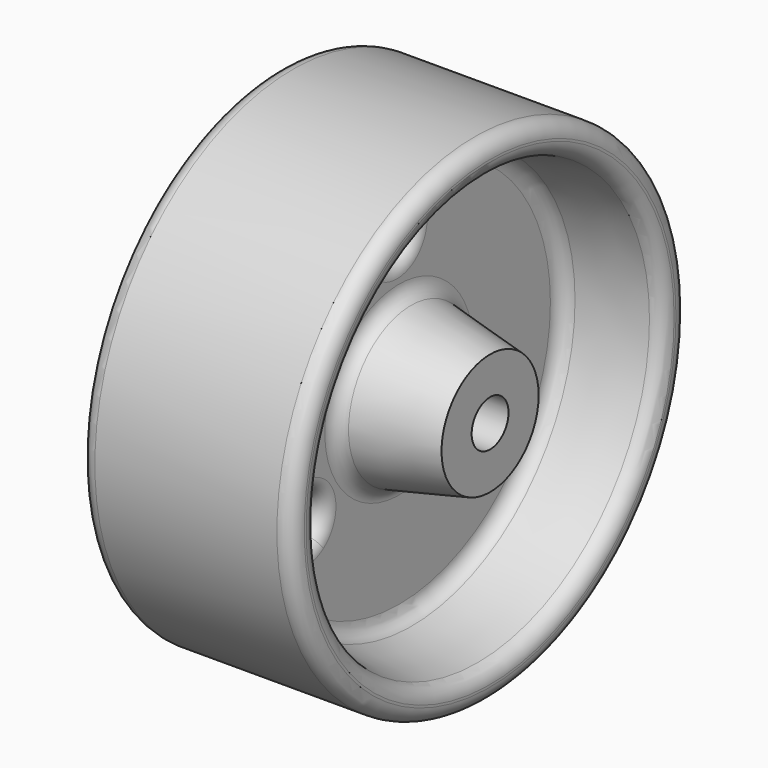
from build123d import *

# Parameters (mm, degrees)
F2_R     = 3.175
F4_DEPTH = 25.4
F5_R     = 3.17499


# Not quite as in the source:
# - a fillet or chamfer is up to 0.001 mm smaller than in the source, because OpenCascade refuses the exact size


with BuildPart() as f1:
    # F0 (on Top) → F1 (revolve)
    with BuildSketch(Plane.XY):
        Polygon((-25.8535725378, 7.874), (-25.8535725378, 0), (24.9464274622, 0), (24.9464274622, 7.874), (5.8964274622, 12.0600205039), (-0.4535725378, 12.0600205039), align=None)
        Polygon((-0.4535725378, 37.4600205039), (-0.4535725378, 12.0600205039), (5.8964274622, 12.0600205039), (5.8964274622, 37.4600205039), (24.9464274622, 40.6350205039), (24.9464274622, 46.9850205039), (-0.4535725378, 46.9850205039), align=None)
        Polygon((-19.5035725378, 40.6350205039), (-0.4535725378, 37.4600205039), (-0.4535725378, 46.9850205039), (-19.5035725378, 46.9850205039), align=None)
    revolve(axis=Axis((-0.2934029948, -4.826, 0), (1, 0, 0)))

    # F2
    f2_edges = [f1.edges().sort_by_distance(p)[0] for p in [
        (5.896427, -47.112021, 0),
        (24.946427, -50.287021, 0),
        (24.946427, -56.637021, 0),
        (5.896427, -21.712021, 0),
        (-19.503573, -56.637021, 0),
        (-19.503573, -50.287021, 0),
        (-0.453573, -21.712021, 0),
        (-0.453573, -47.112021, 0),
    ]]
    fillet(f2_edges, radius=F2_R)

    # F3 (on face) → F4 (cut)
    with BuildSketch(Plane(origin=(-0.4535725378, 0, 0), x_dir=(0, -1, 0), z_dir=(-1, 0, 0))):
        with BuildLine():
            ThreePointArc((0.658709515, 28.2694944244), (5.314152326, 23.8074959531), (10.1485843232, 28.0749126646))
            ThreePointArc((10.1485843232, 28.0749126646), (5.4117827912, 28.5689951437), (0.658709515, 28.2694944244))
        make_face()
        with BuildLine():
            ThreePointArc((0.658709515, 28.2694944244), (5.4117827912, 28.5689951437), (10.1485843232, 28.0749126646))
            ThreePointArc((10.1485843232, 28.0749126646), (10.1678538349, 28.3216199694), (10.1742827912, 28.5689951437))
            ThreePointArc((10.1742827912, 28.5689951437), (5.2619582739, 33.3291378794), (0.658709515, 28.2694944244))
        make_face()
        with BuildLine():
            ThreePointArc((34.0370841595, -14.7918003501), (33.3220764355, -12.2819771442), (31.3917455662, -10.5257677872))
            ThreePointArc((31.3917455662, -10.5257677872), (29.2745841595, -14.7918003501), (26.4782954149, -18.64694957))
            ThreePointArc((26.4782954149, -18.64694957), (31.4383864961, -19.0343662834), (34.0370841595, -14.7918003501))
        make_face()
        with BuildLine():
            ThreePointArc((26.4782954149, -18.64694957), (29.2745841595, -14.7918003501), (31.3917455662, -10.5257677872))
            ThreePointArc((31.3917455662, -10.5257677872), (25.1998201329, -12.3265002918), (26.4782954149, -18.64694957))
        make_face()
        with BuildLine():
            ThreePointArc((-15.4458669506, -13.7771947936), (-17.6160982435, -9.7820040347), (-22.1488797381, -9.4279630946))
            ThreePointArc((-22.1488797381, -9.4279630946), (-20.2083669506, -13.7771947936), (-17.5724550812, -17.7437266372))
            ThreePointArc((-17.5724550812, -17.7437266372), (-16.0110501572, -16.0275143233), (-15.4458669506, -13.7771947936))
        make_face()
        with BuildLine():
            ThreePointArc((-17.5724550812, -17.7437266372), (-20.2083669506, -13.7771947936), (-22.1488797381, -9.4279630946))
            ThreePointArc((-22.1488797381, -9.4279630946), (-24.3807614424, -16.0733939259), (-17.5724550812, -17.7437266372))
        make_face()
    extrude(amount=-F4_DEPTH, mode=Mode.SUBTRACT)

    # F5 (radius 3.175 in the source; OpenCascade refuses exactly that, so slightly less here)
    f5_edges = [f1.edges().sort_by_distance(p)[0] for p in [
        (-0.453573, 18.267854, -18.126426),
        (5.896427, 18.267854, -18.126426),
        (-0.453573, -27.157423, -19.057833),
        (5.896427, -27.157423, -19.057833),
        (-0.453573, -0.674981, 29.063078),
        (5.896427, -0.674981, 29.063078),
    ]]
    fillet(f5_edges, radius=F5_R)


solid = f1.part
